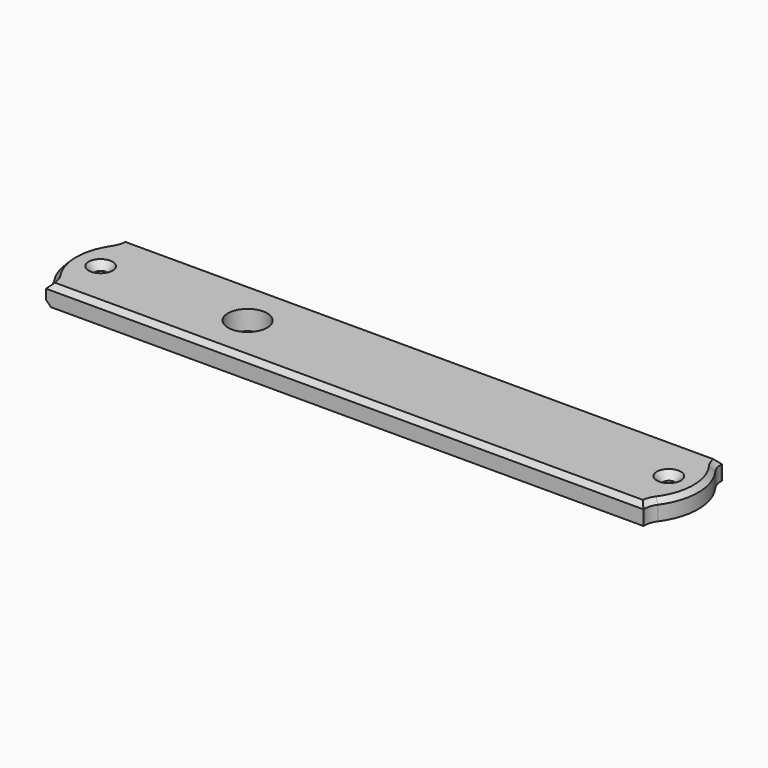
from build123d import *

# Parameters (mm, degrees)
F0_R           = 6.35
F1_DEPTH       = 6.35
F2_D           = 3.7973
F2_CSINK_D     = 7.7978
F2_CSINK_ANGLE = 82
F3_C1_SIZE     = 1.5875
F3_C2_SIZE     = 1.5875
F3_C3_SIZE     = 1.5875
F3_C4_SIZE     = 1.5875
F3_C5_SIZE     = 1.5875


with BuildPart() as f1:
    # F0 (on Top) → F1 (new body)
    with BuildSketch(Plane.XY):
        with BuildLine():
            Line((-87.0919269209, -13.7156903623), (-87.0919269209, -14.792130794))
            Line((-87.0919269209, -14.792130794), (106.5325381816, -14.792130794))
            Line((106.5325381816, -14.792130794), (106.5325381816, -14.3110791923))
            ThreePointArc((106.5325381816, -14.3110791923), (106.846778333, -12.3382378278), (107.7583974098, -10.5606550362))
            ThreePointArc((107.7583974098, -10.5606550362), (111.5641860478, 1.082869206), (107.7583974098, 12.7263934482))
            ThreePointArc((107.7583974098, 12.7263934482), (106.846778333, 14.5039762398), (106.5325381816, 16.4768176043))
            Line((106.5325381816, 16.4768176043), (106.5325381816, 16.957869206))
            Line((106.5325381816, 16.957869206), (-87.0919269209, 16.957869206))
            Line((-87.0919269209, 16.957869206), (-87.0919269209, 15.8814287743))
            ThreePointArc((-87.0919269209, 15.8814287743), (-87.3716340972, 14.0175497454), (-88.1861143334, 12.3178723984))
            ThreePointArc((-88.1861143334, 12.3178723984), (-91.6358139522, 1.082869206), (-88.1861143334, -10.1521339864))
            ThreePointArc((-88.1861143334, -10.1521339864), (-87.3716340972, -11.8518113334), (-87.0919269209, -13.7156903623))
        make_face()
        with Locations((-34.4858139522, 1.082869206)):
            Circle(F0_R, mode=Mode.SUBTRACT)
    extrude(amount=-F1_DEPTH)

    # F2 (through all)
    with Locations(Plane.XY):
        with Locations((102.0391860478, 1.082869206), (-82.1108139522, 1.082869206)):
            CounterSinkHole(F2_D / 2, F2_CSINK_D / 2, counter_sink_angle=F2_CSINK_ANGLE)

    # F3: chamfer of 1.5875 on 9 edges, made by hand

    # F3_c1
    f3_c1_edges = [f1.edges().sort_by_distance(p)[0] for p in [
        (-87.3716340972, -11.8518113334, 0),
        (-91.6358139522, 1.082869206, 0),
        (-87.0919269209, -14.2539105781, 0),
        (-87.3716340972, 14.0175497454, 0),
        (-87.0919269209, 16.4196489902, 0),
    ]]
    chamfer(f3_c1_edges, length=F3_C1_SIZE)

    # F3_c2
    f3_c2_edges = [f1.edges().sort_by_distance(p)[0] for p in [
        (-87.3716340972, -11.8518113334, -6.35),
        (-91.6358139522, 1.082869206, -6.35),
        (-87.0919269209, -14.2539105781, -6.35),
        (-87.3716340972, 14.0175497454, -6.35),
        (-87.0919269209, 16.4196489902, -6.35),
    ]]
    chamfer(f3_c2_edges, length=F3_C2_SIZE)

    # F3_c3
    f3_c3_edges = [f1.edges().sort_by_distance(p)[0] for p in [
        (106.5325381816, -14.5516049932, 0),
        (106.846778333, -12.3382378278, 0),
        (106.5325381816, 16.7173434052, 0),
        (111.5641860478, 1.082869206, 0),
        (106.846778333, 14.5039762398, 0),
    ]]
    chamfer(f3_c3_edges, length=F3_C3_SIZE)

    # F3_c4
    f3_c4_edges = [f1.edges().sort_by_distance(p)[0] for p in [
        (9.7203056303, -14.792130794, 0),
    ]]
    chamfer(f3_c4_edges, length=F3_C4_SIZE)

    # F3_c5
    f3_c5_edges = [f1.edges().sort_by_distance(p)[0] for p in [
        (9.7203056303, 16.957869206, 0),
    ]]
    chamfer(f3_c5_edges, length=F3_C5_SIZE)


solid = f1.part
